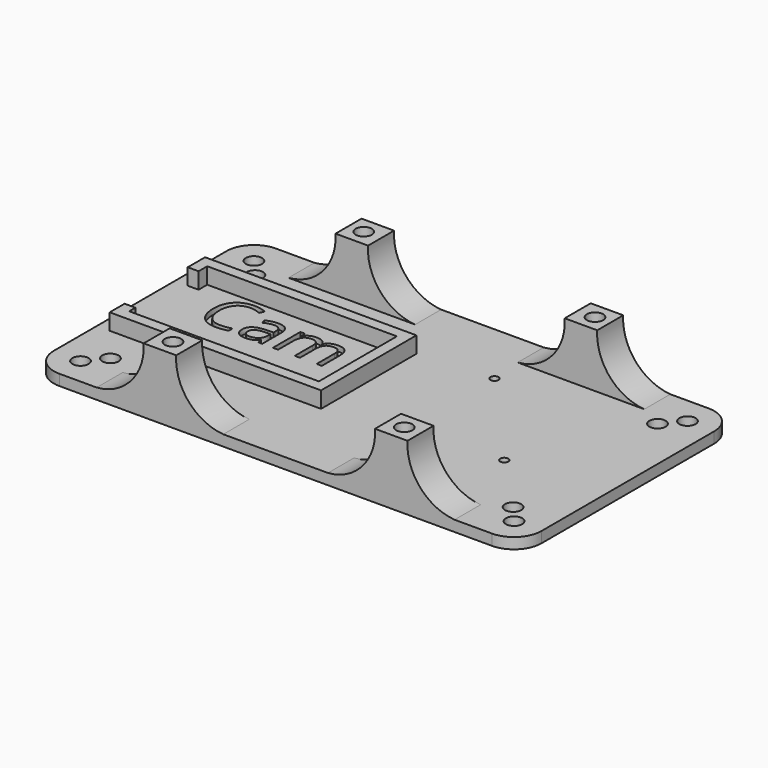
from build123d import *

# Parameters (mm, degrees)
F0_W          = 90
F0_H          = 50
F1_DEPTH      = 2
F3_R          = 5.08
F4_R          = 5.08
F5_R          = 5.08
F6_R          = 5.08
F8_R          = 1.5
F9_DEPTH      = 25.4
F10_R         = 0.75
F11_DEPTH     = 25.4
F12_TEXT_SIZE = 11.8391950511
F13_DEPTH     = 1
F15_DEPTH     = 3
F18_DEPTH     = 6
F22_DEPTH     = 6
F23_R         = 1.5
F24_DEPTH     = 10


# Not quite as in the source:
# - Text() gives the source's letters only with a copy of the font that has no kerning and outlines rounded to 1/6400 em; it was checked with that copy


with BuildPart() as f1:
    # F0 (on Top) → F1 (new body)
    with BuildSketch(Plane.XY):
        with Locations((45, 25)):
            Rectangle(F0_W, F0_H)
    extrude(amount=F1_DEPTH)

    # F3
    f3_edges = [f1.edges().sort_by_distance(p)[0] for p in [
        (90, 0, 1),
    ]]
    fillet(f3_edges, radius=F3_R)

    # F4
    f4_edges = [f1.edges().sort_by_distance(p)[0] for p in [
        (90, 50, 1),
    ]]
    fillet(f4_edges, radius=F4_R)

    # F5
    f5_edges = [f1.edges().sort_by_distance(p)[0] for p in [
        (0, 50, 1),
    ]]
    fillet(f5_edges, radius=F5_R)

    # F6
    f6_edges = [f1.edges().sort_by_distance(p)[0] for p in [
        (0, 0, 1),
    ]]
    fillet(f6_edges, radius=F6_R)

    # F8 (on offset) → F9 (cut)
    with BuildSketch(Plane.XY.offset(2)):
        with Locations((85, 5)):
            Circle(F8_R)
        with Locations((82.1494022449, 8.3385913854)):
            Circle(F8_R)
        with Locations((82.1494022449, 41.6614086146)):
            Circle(F8_R)
        with Locations((85, 45)):
            Circle(F8_R)
        with Locations((7.8505977551, 41.6614086146)):
            Circle(F8_R)
        with Locations((5, 45)):
            Circle(F8_R)
        with Locations((7.8505977551, 8.3385913854)):
            Circle(F8_R)
        with Locations((5, 5)):
            Circle(F8_R)
    extrude(amount=-F9_DEPTH, mode=Mode.SUBTRACT)

    # F10 (on offset) → F11 (cut)
    with BuildSketch(Plane.XY.offset(2)):
        with Locations((72, 19)):
            Circle(F10_R)
        with Locations((55, 38)):
            Circle(F10_R)
    extrude(amount=-F11_DEPTH, mode=Mode.SUBTRACT)

    # F12 (on offset) → F13 (cut)
    with BuildSketch(Plane.XY.offset(2)):
        with Locations((8.9907050133, 25.5434624851)):
            Text('Cam', F12_TEXT_SIZE, font='Open Sans', text_align=(TextAlign.LEFT, TextAlign.BOTTOM))
    extrude(amount=-F13_DEPTH, mode=Mode.SUBTRACT)

    # F14 (on offset) → F15 (join)
    with BuildSketch(Plane.XY.offset(2)):
        Polygon((4.3826700747, 33), (4.3826700747, 35), (39.3826700747, 35), (39.3826700747, 17), (4.3826700747, 17), (4.3826700747, 18.4396387637), (2.3826700747, 18.4396387637), (2.3826700747, 15), (41.3826700747, 15), (41.3826700747, 37), (2.3826700747, 37), (2.3826700747, 33), align=None)
    extrude(amount=F15_DEPTH)

    # F17 (on offset) → F18 (join)
    with BuildSketch(Plane.XZ):
        with BuildLine():
            Line((11.9775680869, 2), (10.5156, 2))
            ThreePointArc((10.5156, 2), (11.2465840435, 1.9716326499), (11.9775680869, 2))
        make_face()
        with BuildLine():
            Line((36.8046, 2), (35.3426319131, 2))
            ThreePointArc((35.3426319131, 2), (36.0736159565, 1.9716326499), (36.8046, 2))
        make_face()
        with BuildLine():
            ThreePointArc((20.6601, 12), (18.3689235511, 5.2200032425), (11.9775680869, 2))
            Line((11.9775680869, 2), (23.6601, 2))
            Line((23.6601, 2), (23.6601, 12))
            Line((23.6601, 12), (20.6601, 12))
        make_face()
        with BuildLine():
            Line((23.6601, 12), (23.6601, 2))
            Line((23.6601, 2), (35.3426319131, 2))
            ThreePointArc((35.3426319131, 2), (28.9512764489, 5.2200032425), (26.6601, 12))
            Line((26.6601, 12), (23.6601, 12))
        make_face()
        with BuildLine():
            Line((54.6573680869, 2), (53.1954, 2))
            ThreePointArc((53.1954, 2), (53.9263840435, 1.9716326499), (54.6573680869, 2))
        make_face()
        with BuildLine():
            Line((79.4844, 2), (78.0224319131, 2))
            ThreePointArc((78.0224319131, 2), (78.7534159565, 1.9716326499), (79.4844, 2))
        make_face()
        with BuildLine():
            ThreePointArc((63.3399, 12), (61.0487235511, 5.2200032425), (54.6573680869, 2))
            Line((54.6573680869, 2), (78.0224319131, 2))
            ThreePointArc((78.0224319131, 2), (71.6310764489, 5.2200032425), (69.3399, 12))
            Line((69.3399, 12), (63.3399, 12))
        make_face()
    extrude(amount=-F18_DEPTH)

    # F21 (on offset) → F22 (join)
    with BuildSketch(Plane(origin=(0, 50, 0), x_dir=(-1, 0, 0), z_dir=(0, 1, 0))):
        with BuildLine():
            Line((-77.8270319131, 2), (-79.289, 2))
            ThreePointArc((-79.289, 2), (-78.5580159565, 1.9716326499), (-77.8270319131, 2))
        make_face()
        with BuildLine():
            Line((-53, 2), (-54.4619680869, 2))
            ThreePointArc((-54.4619680869, 2), (-53.7309840435, 1.9716326499), (-53, 2))
        make_face()
        with BuildLine():
            ThreePointArc((-69.1445, 12), (-71.4356764489, 5.2200032425), (-77.8270319131, 2))
            Line((-77.8270319131, 2), (-66.1445, 2))
            Line((-66.1445, 2), (-66.1445, 12))
            Line((-66.1445, 12), (-69.1445, 12))
        make_face()
        with BuildLine():
            Line((-66.1445, 12), (-66.1445, 2))
            Line((-66.1445, 2), (-54.4619680869, 2))
            ThreePointArc((-54.4619680869, 2), (-60.8533235511, 5.2200032425), (-63.1445, 12))
            Line((-63.1445, 12), (-66.1445, 12))
        make_face()
        with BuildLine():
            Line((-35.5380319131, 2), (-37, 2))
            ThreePointArc((-37, 2), (-36.2690159565, 1.9716326499), (-35.5380319131, 2))
        make_face()
        with BuildLine():
            Line((-10.711, 2), (-12.1729680869, 2))
            ThreePointArc((-12.1729680869, 2), (-11.4419840435, 1.9716326499), (-10.711, 2))
        make_face()
        with BuildLine():
            ThreePointArc((-26.8555, 12), (-29.1466764489, 5.2200032425), (-35.5380319131, 2))
            Line((-35.5380319131, 2), (-12.1729680869, 2))
            ThreePointArc((-12.1729680869, 2), (-18.5643235511, 5.2200032425), (-20.8555, 12))
            Line((-20.8555, 12), (-26.8555, 12))
        make_face()
    extrude(amount=-F22_DEPTH)

    # F23 (on offset) → F24 (cut)
    with BuildSketch(Plane.XY.offset(12)):
        with Locations((23.6601, 3)):
            Circle(F23_R)
        with Locations((66.3399, 3)):
            Circle(F23_R)
        with Locations((23.6601, 47)):
            Circle(F23_R)
        with Locations((66.3399, 47)):
            Circle(F23_R)
    extrude(amount=-F24_DEPTH, mode=Mode.SUBTRACT)


solid = f1.part
